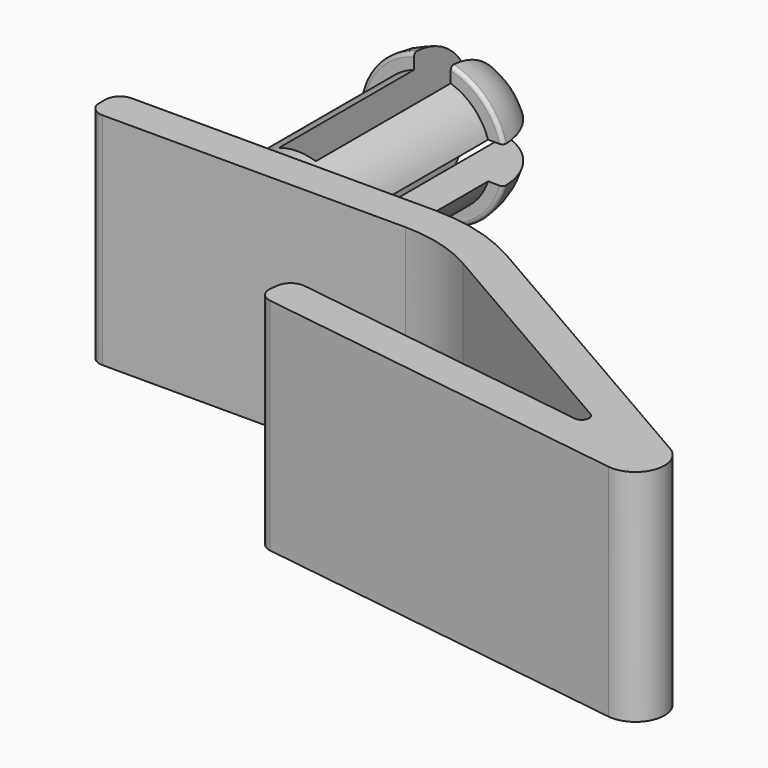
from build123d import *

# Parameters (mm, degrees)
F1_DEPTH  = 7.62
F3_W      = 0.635
F3_H      = 5.842
F6_DEPTH  = 12.7
F7_R      = 0.127
F9_W      = 10.16
F9_H      = 1.27
F10_DEPTH = 3.175


with BuildPart() as f1:
    # F0 (on Top) → F1 (new body)
    with BuildSketch(Plane.XY):
        with BuildLine():
            Line((10.9985226281, 0), (0.508, 0))
            ThreePointArc((0.508, 0), (0.1487897552, -0.1487897552), (0, -0.508))
            Line((0, -0.508), (0, -0.762))
            ThreePointArc((0, -0.762), (0.1487897552, -1.1212102448), (0.508, -1.27))
            Line((0.508, -1.27), (10.9985226281, -1.27))
            ThreePointArc((10.9985226281, -1.27), (12.3133233772, -1.4430968025), (13.5385226281, -1.9505909488))
            Line((13.5385226281, -1.9505909488), (21.7479125756, -6.6902844449))
            ThreePointArc((21.7479125756, -6.6902844449), (21.8610174728, -6.9931140452), (21.5852173248, -7.1617342188))
            Line((21.5852173248, -7.1617342188), (11.0182697374, -5.6618500829))
            ThreePointArc((11.0182697374, -5.6618500829), (10.6417144767, -5.7586825509), (10.4439205931, -6.093418224))
            Line((10.4439205931, -6.093418224), (10.4082253422, -6.3448975453))
            ThreePointArc((10.4082253422, -6.3448975453), (10.5050578102, -6.7214528061), (10.8397934833, -6.9192466897))
            Line((10.8397934833, -6.9192466897), (24.0516598784, -8.7945535034))
            ThreePointArc((24.0516598784, -8.7945535034), (25.144685653, -8.1262935433), (24.6964387295, -6.9261471298))
            Line((24.6964387295, -6.9261471298), (14.1735226281, -0.850738686))
            ThreePointArc((14.1735226281, -0.850738686), (12.6420235645, -0.2163710031), (10.9985226281, 0))
        make_face()
    extrude(amount=F1_DEPTH)

    # F3 (on offset) → F4 (revolve)
    with BuildSketch(Plane.XY.offset(3.81)):
        Polygon((3.81, 3.048), (3.81, 0), (5.842, 0), (5.842, 8.89), (4.445, 8.89), (4.445, 3.048), align=None)
        with BuildLine():
            Line((4.445, 8.89), (5.842, 8.89))
            Line((5.842, 8.89), (6.35, 8.89))
            ThreePointArc((6.35, 8.89), (5.8180463142, 10.4454259867), (4.445, 11.3493444248))
            Line((4.445, 11.3493444248), (4.445, 8.89))
        make_face()
        with BuildLine():
            Line((3.81, 11.43), (3.81, 8.89))
            Line((3.81, 8.89), (4.445, 8.89))
            Line((4.445, 8.89), (4.445, 11.3493444248))
            ThreePointArc((4.445, 11.3493444248), (4.1300509029, 11.4097554285), (3.81, 11.43))
        make_face()
        with Locations((4.1275, 5.969)):
            Rectangle(F3_W, F3_H)
    revolve(axis=Axis((3.81, 4.445, 3.81), (0, 1, 0)))

    # F5 (on offset) → F6 (cut, symmetric)
    with BuildSketch(Plane.XY.offset(3.81)):
        Polygon((3.175, 3.048), (3.81, 3.048), (4.445, 3.048), (4.445, 13.208), (3.175, 13.208), align=None)
    extrude(amount=F6_DEPTH, both=True, mode=Mode.SUBTRACT)

    # F7
    f7_edges = [f1.edges().sort_by_distance(p)[0] for p in [
        (1.27, 8.89, 3.81),
        (6.35, 8.89, 3.81),
    ]]
    fillet(f7_edges, radius=F7_R)

    # F9 (on offset) → F10 (cut, symmetric)
    with BuildSketch(Plane(origin=(3.81, 0, 0), x_dir=(0, -1, 0), z_dir=(-1, 0, 0))):
        with Locations((-8.128, 3.81)):
            Rectangle(F9_W, F9_H)
    extrude(amount=F10_DEPTH, both=True, mode=Mode.SUBTRACT)


solid = f1.part
